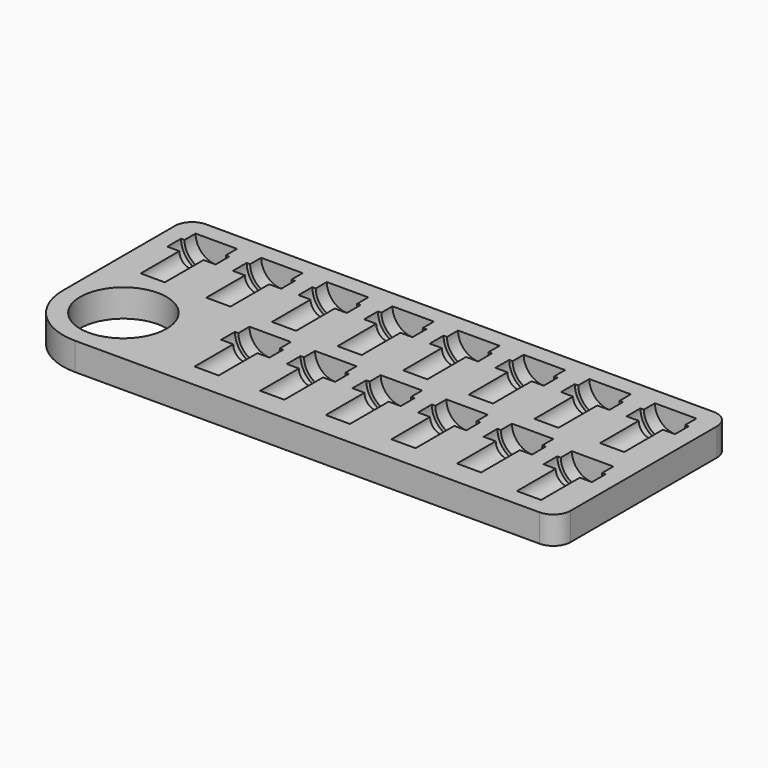
from build123d import *

# Parameters (mm, degrees)
F0_R          = 12.5
F1_DEPTH      = 8
F11_TEXT_SIZE = 5.5555555556
F12_DEPTH     = 1


# Not quite as in the source:
# - Text() gives the source's letters only with a copy of the font that has no kerning and outlines rounded to 1/6400 em; it was checked with that copy


with BuildPart() as f1:
    # F0 (on Top) → F1 (new body)
    with BuildSketch(Plane.XY):
        with BuildLine():
            ThreePointArc((0, 17.5), (5.1256313292, 5.1256313292), (17.5, 0))
            Line((17.5, 0), (152, 0))
            ThreePointArc((152, 0), (155.5355339059, 1.4644660941), (157, 5))
            Line((157, 5), (157, 58))
            ThreePointArc((157, 58), (155.5355339059, 61.5355339059), (152, 63))
            Line((152, 63), (5, 63))
            ThreePointArc((5, 63), (1.4644660941, 61.5355339059), (0, 58))
            Line((0, 58), (0, 17.5))
        make_face()
        with Locations((17.5, 17.5)):
            Circle(F0_R, mode=Mode.SUBTRACT)
    extrude(amount=F1_DEPTH)

    # F2 (on face) → F3 (revolve, cut)
    with BuildSketch(Plane.XY.offset(8)):
        Polygon((12, 49), (12, 35), (15.5, 35), (15.5, 49), (19, 49), (19, 54), (18, 54), (18, 58), (12, 58), (12, 54), align=None)
    revolve(axis=Axis((12, 42, 8), (0, 1, 0)), mode=Mode.SUBTRACT)

    # F2 (on face) → F4 (revolve, cut)
    with BuildSketch(Plane.XY.offset(8)):
        Polygon((31, 49), (31, 35), (34.5, 35), (34.5, 49), (38, 49), (38, 54), (37, 54), (37, 58), (31, 58), (31, 54), align=None)
    revolve(axis=Axis((31, 42, 8), (0, 1, 0)), mode=Mode.SUBTRACT)

    # F2 (on face) → F5 (revolve, cut)
    with BuildSketch(Plane.XY.offset(8)):
        Polygon((50, 21), (50, 7), (53.5, 7), (53.5, 21), (57, 21), (57, 26), (56, 26), (56, 30), (50, 30), (50, 26), align=None)
        Polygon((50, 49), (50, 35), (53.5, 35), (53.5, 49), (57, 49), (57, 54), (56, 54), (56, 58), (50, 58), (50, 54), align=None)
    revolve(axis=Axis((50, 42, 8), (0, 1, 0)), mode=Mode.SUBTRACT)

    # F2 (on face) → F6 (revolve, cut)
    with BuildSketch(Plane.XY.offset(8)):
        Polygon((69, 21), (69, 7), (72.5, 7), (72.5, 21), (76, 21), (76, 26), (75, 26), (75, 30), (69, 30), (69, 26), align=None)
        Polygon((69, 49), (69, 35), (72.5, 35), (72.5, 49), (76, 49), (76, 54), (75, 54), (75, 58), (69, 58), (69, 54), align=None)
    revolve(axis=Axis((69, 42, 8), (0, 1, 0)), mode=Mode.SUBTRACT)

    # F2 (on face) → F7 (revolve, cut)
    with BuildSketch(Plane.XY.offset(8)):
        Polygon((88, 21), (88, 7), (91.5, 7), (91.5, 21), (95, 21), (95, 26), (94, 26), (94, 30), (88, 30), (88, 26), align=None)
        Polygon((88, 49), (88, 35), (91.5, 35), (91.5, 49), (95, 49), (95, 54), (94, 54), (94, 58), (88, 58), (88, 54), align=None)
    revolve(axis=Axis((88, 42, 8), (0, 1, 0)), mode=Mode.SUBTRACT)

    # F2 (on face) → F8 (revolve, cut)
    with BuildSketch(Plane.XY.offset(8)):
        Polygon((107, 21), (107, 7), (110.5, 7), (110.5, 21), (114, 21), (114, 26), (113, 26), (113, 30), (107, 30), (107, 26), align=None)
        Polygon((107, 49), (107, 35), (110.5, 35), (110.5, 49), (114, 49), (114, 54), (113, 54), (113, 58), (107, 58), (107, 54), align=None)
    revolve(axis=Axis((107, 42, 8), (0, 1, 0)), mode=Mode.SUBTRACT)

    # F2 (on face) → F9 (revolve, cut)
    with BuildSketch(Plane.XY.offset(8)):
        Polygon((126, 21), (126, 7), (129.5, 7), (129.5, 21), (133, 21), (133, 26), (132, 26), (132, 30), (126, 30), (126, 26), align=None)
        Polygon((126, 49), (126, 35), (129.5, 35), (129.5, 49), (133, 49), (133, 54), (132, 54), (132, 58), (126, 58), (126, 54), align=None)
    revolve(axis=Axis((126, 42, 8), (0, 1, 0)), mode=Mode.SUBTRACT)

    # F2 (on face) → F10 (revolve, cut)
    with BuildSketch(Plane.XY.offset(8)):
        Polygon((145, 18.9371687499), (145, 4.9371687499), (148.5, 4.9371687499), (148.5, 18.9371687499), (152, 18.9371687499), (152, 23.9371687499), (151, 23.9371687499), (151, 27.9371687499), (145, 27.9371687499), (145, 23.9371687499), align=None)
        Polygon((145, 49), (145, 35), (148.5, 35), (148.5, 49), (152, 49), (152, 54), (151, 54), (151, 58), (145, 58), (145, 54), align=None)
    revolve(axis=Axis((145, 42, 8), (0, 1, 0)), mode=Mode.SUBTRACT)

    # F11 (on face) → F12 (cut)
    with BuildSketch(Plane(origin=(0, 0, 0), x_dir=(1, 0, 0), z_dir=(0, 0, -1))):
        with Locations((30, -9)):
            Text('874, 875', F11_TEXT_SIZE, font='Open Sans', text_align=(TextAlign.LEFT, TextAlign.BOTTOM))
    extrude(amount=-F12_DEPTH, mode=Mode.SUBTRACT)


solid = f1.part
